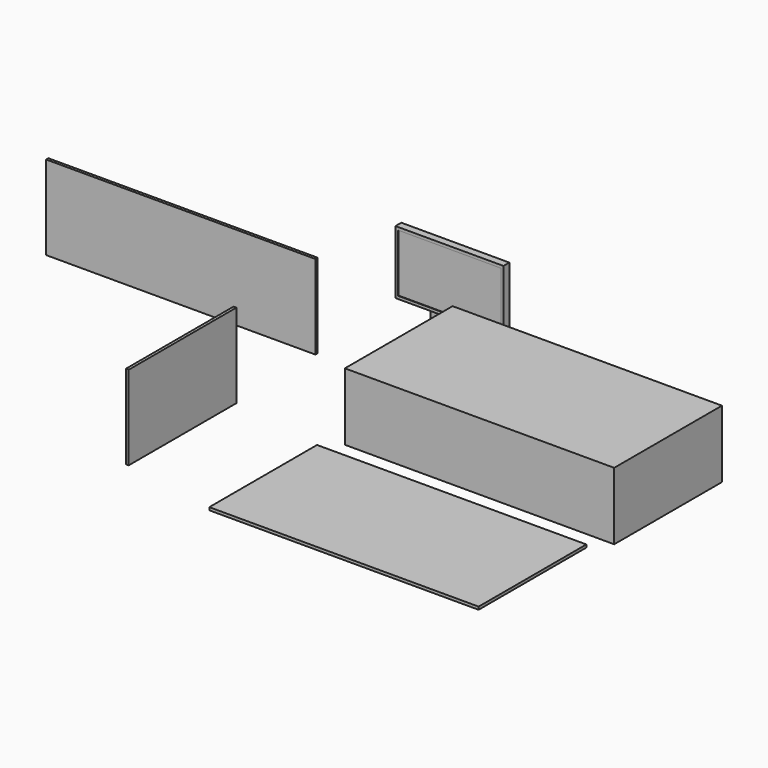
from build123d import *

# Parameters (mm, degrees)
F1_W      = 977.9
F1_H      = 574.04
F2_DEPTH  = 66.04
F3_W      = 929.64
F3_H      = 523.24
F4_DEPTH  = 5.08
F5_W      = 2438.4
F5_H      = 1219.2
F6_DEPTH  = 609.6
F7_W      = 2438.4
F7_H      = 1219.2
F8_DEPTH  = 25.4
F9_W      = 2438.4
F9_H      = 762
F10_DEPTH = 25.4
F11_W     = 1219.2
F11_H     = 762
F12_DEPTH = 25.4
F13_W     = 406.4
F13_H     = 152.4
F14_DEPTH = 640.08
F15_SIZE2 = 87.988171
F15_SIZE  = 152.39999


# Not quite as in the source:
# - a fillet or chamfer is up to 0.001 mm smaller than in the source, because OpenCascade refuses the exact size


with BuildPart() as f2:
    # F1 (on Front) → F2 (new body)
    with BuildSketch(Plane.XZ):
        with Locations((554.5943079948, 565.9104996113)):
            Rectangle(F1_W, F1_H)
    extrude(amount=F2_DEPTH)

    # F3 (on face) → F4 (cut)
    with BuildSketch(Plane.XZ.offset(66.04)):
        with Locations((554.5943079948, 565.9104996113)):
            Rectangle(F3_W, F3_H)
    extrude(amount=-F4_DEPTH, mode=Mode.SUBTRACT)


with BuildPart() as f6:
    # F5 (on face) → F6 (new body)
    with BuildSketch(Plane.XY):
        with Locations((2074.7481584549, -1016.0588382279)):
            Rectangle(F5_W, F5_H)
    extrude(amount=F6_DEPTH)


with BuildPart() as f8:
    # F7 (on face) → F8 (new body)
    with BuildSketch(Plane.XY):
        with Locations((1952.8129696846, -2398.0931629392)):
            Rectangle(F7_W, F7_H)
    extrude(amount=F8_DEPTH)


with BuildPart() as f10:
    # F9 (on Front) → F10 (new body)
    with BuildSketch(Plane.XZ):
        with Locations((-1910.7732921839, -53.4418959455)):
            Rectangle(F9_W, F9_H)
    extrude(amount=F10_DEPTH)


with BuildPart() as f12:
    # F11 (on Right) → F12 (new body)
    with BuildSketch(Plane.YZ):
        with Locations((-2425.0782728195, 519.9815827243)):
            Rectangle(F11_W, F11_H)
    extrude(amount=F12_DEPTH)


with BuildPart() as f14:
    # F13 (on face) → F14 (new body)
    with BuildSketch(Plane.XY):
        with Locations((514.7094428539, 99.033133836)):
            Rectangle(F13_W, F13_H)
    extrude(amount=F14_DEPTH)

    # F15 (size 152.4 and 87.9881810245 in the source; OpenCascade refuses exactly that, so slightly less here)
    f15_edges = [f14.edges().sort_by_distance(p)[0] for p in [
        (514.709443, 175.233134, 640.08),
    ]]
    f15_side = f14.faces().sort_by_distance((514.709443, 99.033134, 640.08))[0]
    chamfer(f15_edges, length=F15_SIZE, length2=F15_SIZE2, reference=f15_side)


solid = Compound([f2.part, f6.part, f8.part, f10.part, f12.part, f14.part])
